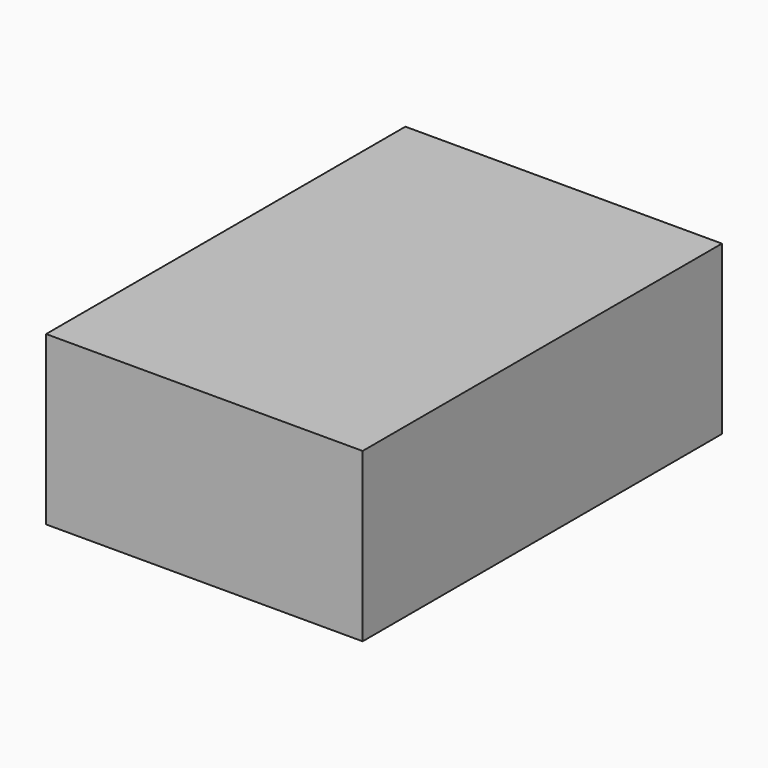
from build123d import *

# Parameters (mm, degrees)
F0_W     = 50.1842871308
F0_H     = 26.5729175881
F1_DEPTH = 25
F2_DEPTH = 71.2


# Not quite as in the source:
# - the program builds the solid bodies; features that only make, move or delete a surface that nothing else refers to are left out


with BuildPart() as f1:
    # F0 (on Front) → F1 (new body)
    with BuildSketch(Plane.XZ):
        with Locations((54.8890642822, 5.7227066718)):
            Rectangle(F0_W, F0_H)
    extrude(amount=F1_DEPTH)

    # F0 (on Front) → F2 (join)
    with BuildSketch(Plane.XZ):
        with Locations((54.8890642822, 5.7227066718)):
            Rectangle(F0_W, F0_H)
    extrude(amount=F2_DEPTH)


solid = f1.part
